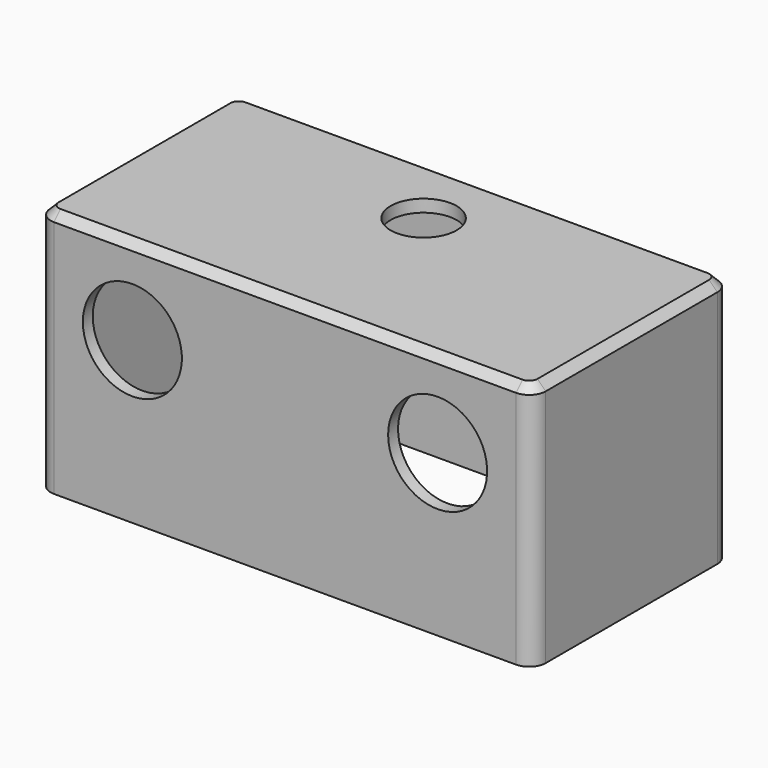
from build123d import *

# Parameters (mm, degrees)
F0_W     = 60
F0_H     = 30
F1_DEPTH = 30
F2_T     = -1.5
F3_R     = 6
F4_DEPTH = 1.501
F5_R     = 4
F6_DEPTH = 30.001
F7_R     = 2
F8_SIZE  = 1


with BuildPart() as f1:
    # F0 (on Top) → F1 (new body)
    with BuildSketch(Plane.XY):
        Rectangle(F0_W, F0_H)
    extrude(amount=F1_DEPTH)

    # F2
    f2_openings = [f1.faces().sort_by_distance(p)[0] for p in [
        (0, 0, 0),
    ]]
    offset(amount=F2_T, openings=f2_openings)

    # F3 (on face) → F4 (cut, through all)
    with BuildSketch(Plane(origin=(0, -13.5, 0), x_dir=(-1, 0, 0), z_dir=(0, 1, 0))):
        with Locations((-18.5, 19.5)):
            Circle(F3_R)
        with Locations((18.5, 19.5)):
            Circle(F3_R)
    extrude(amount=-F4_DEPTH, mode=Mode.SUBTRACT)

    # F5 (on face) → F6 (cut, through all)
    with BuildSketch(Plane.XY.offset(30)):
        with Locations((0, 6)):
            Circle(F5_R)
    extrude(amount=-F6_DEPTH, mode=Mode.SUBTRACT)

    # F7
    f7_edges = [f1.edges().sort_by_distance(p)[0] for p in [
        (30, 15, 15),
        (30, -15, 15),
        (-30, -15, 15),
        (-30, 15, 15),
    ]]
    fillet(f7_edges, radius=F7_R)

    # F8
    f8_edges = [f1.edges().sort_by_distance(p)[0] for p in [
        (28.5, 0, 28.5),
        (0, 13.5, 28.5),
        (0, -13.5, 28.5),
        (-28.5, 0, 28.5),
        (28.5, -13.5, 14.25),
        (28.5, 13.5, 14.25),
        (-28.5, -13.5, 14.25),
        (-28.5, 13.5, 14.25),
        (0, 15, 30),
        (30, 0, 30),
        (-30, 0, 30),
        (0, -15, 30),
    ]]
    chamfer(f8_edges, length=F8_SIZE)


solid = f1.part
